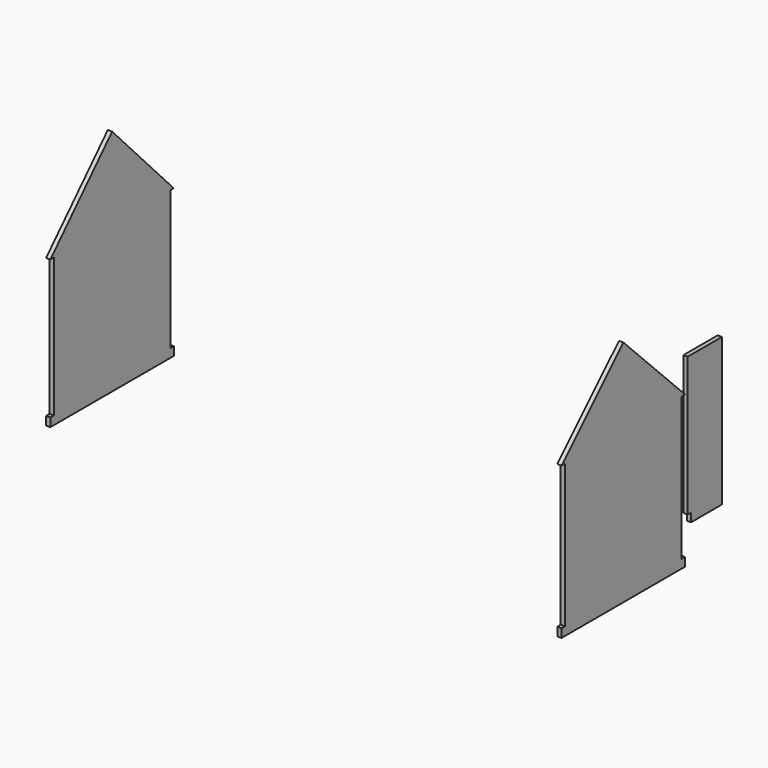
from build123d import *

# Parameters (mm, degrees)
F1_DEPTH = 1
F2_DEPTH = 1
F0_W     = 1
F0_H     = 2
F3_DEPTH = 1


with BuildPart() as f1:
    # F0 (on Right) → F1 (new body)
    with BuildSketch(Plane.YZ):
        Polygon((53.3996237096, 51.2606592213), (35.3996237096, 69.2606592213), (17.3996237096, 51.2606592213), (18.3996237096, 51.2606592213), (18.3996237096, 26.2606592213), (18.3996237096, 17.8606592213), (17.3996237096, 17.8606592213), (17.3996237096, 15.8606592213), (53.3996237096, 15.8606592213), (53.3996237096, 17.8606592213), (52.3996237096, 17.8606592213), (52.3996237096, 24.2606592213), (52.3996237096, 26.2606592213), (52.3996237096, 51.2606592213), align=None)
    extrude(amount=F1_DEPTH)


with BuildPart() as f1b:
    # F0 (on Right) → F1, piece 2 (new body)
    with BuildSketch(Plane.YZ):
        Polygon((55.1692863107, 26.2606592213), (55.1692863107, 24.2606592213), (62.1692863107, 24.2606592213), (64.1692863107, 24.2606592213), (64.1692863107, 58.6886592213), (62.1692863107, 58.6886592213), (54.1692863107, 58.6886592213), (54.1692863107, 56.6886592213), (54.1692863107, 26.2606592213), align=None)
    extrude(amount=F1_DEPTH)


with BuildPart() as f1c:
    # F0 (on Right) → F1, piece 3 (new body)
    with BuildSketch(Plane.YZ):
        Polygon((-113.677120924, 154.1882742229), (-130.677120924, 154.1882742229), (-130.677120924, 121.7591796517), (-130.677120924, 119.7591796517), (-113.677120924, 119.7591796517), align=None)
    extrude(amount=F1_DEPTH)

    # F0 (on Right) → F2 (join)
    with BuildSketch(Plane.YZ):
        Polygon((-96.677120924, 154.1882742229), (-113.677120924, 154.1882742229), (-113.677120924, 119.7591796517), (-96.677120924, 119.7591796517), (-96.677120924, 121.7591796517), align=None)
        Polygon((-95.677120924, 154.1882742229), (-113.677120924, 173.1591796517), (-113.677120924, 154.1882742229), (-96.677120924, 154.1882742229), align=None)
        Polygon((-113.677120924, 173.1591796517), (-131.677120924, 154.1882742229), (-130.677120924, 154.1882742229), (-113.677120924, 154.1882742229), align=None)
        Polygon((-113.677120924, 154.1882742229), (-130.677120924, 154.1882742229), (-130.677120924, 121.7591796517), (-130.677120924, 119.7591796517), (-113.677120924, 119.7591796517), align=None)
    extrude(amount=F2_DEPTH)

    # F0 (on Right) → F3 (join)
    with BuildSketch(Plane.YZ):
        with Locations((-131.177120924, 120.7591796517)):
            Rectangle(F0_W, F0_H)
        with Locations((-96.177120924, 120.7591796517)):
            Rectangle(F0_W, F0_H)
    extrude(amount=F3_DEPTH)


solid = Compound([f1.part, f1b.part, f1c.part])
